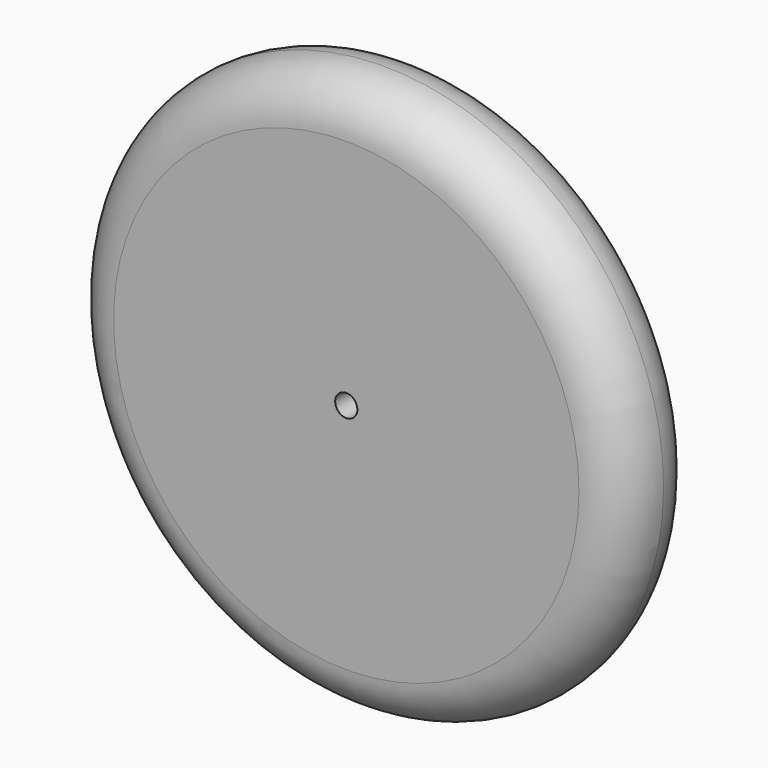
from build123d import *

# Parameters (mm, degrees)
F0_R     = 37.7825
F1_DEPTH = 12.7
F2_R     = 6.35
F3_R     = 6.34999
F4_R     = 1.4986
F5_DEPTH = 12.701


# Not quite as in the source:
# - a fillet or chamfer is up to 0.001 mm smaller than in the source, because OpenCascade refuses the exact size


with BuildPart() as f1:
    # F0 (on Front) → F1 (new body)
    with BuildSketch(Plane.XZ):
        with Locations((-56.96824193, 43.9220815897)):
            Circle(F0_R)
    extrude(amount=F1_DEPTH)

    # F2
    f2_edges = [f1.edges().sort_by_distance(p)[0] for p in [
        (-94.750742, -12.7, 43.922082),
    ]]
    fillet(f2_edges, radius=F2_R)

    # F3 (radius 6.35 in the source; OpenCascade refuses exactly that, so slightly less here)
    f3_edges = [f1.edges().sort_by_distance(p)[0] for p in [
        (-94.750742, 0, 43.922082),
    ]]
    fillet(f3_edges, radius=F3_R)

    # F4 (on face) → F5 (cut, through all)
    with BuildSketch(Plane.XZ.offset(12.7)):
        with Locations((-56.96824193, 43.9220815897)):
            Circle(F4_R)
    extrude(amount=-F5_DEPTH, mode=Mode.SUBTRACT)


solid = f1.part
